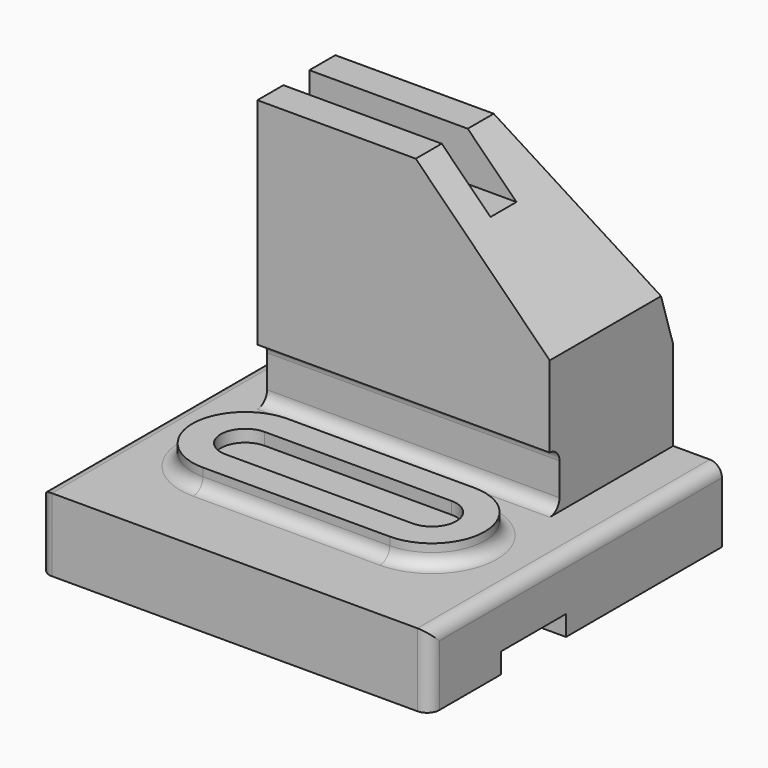
from build123d import *

# Parameters (mm, degrees)
F0_W      = 96
F0_H      = 90
F1_DEPTH  = 18
F2_W      = 72
F2_H      = 38
F4_DEPTH  = 67
F6_DEPTH  = 38
F7_W      = 8
F7_H      = 12
F8_DEPTH  = 51.001
F10_DEPTH = 72.001
F11_W     = 20
F11_H     = 5
F12_DEPTH = 96
F13_W     = 46
F13_H     = 26
F14_DEPTH = 5
F16_DEPTH = 3
F17_W     = 3
F17_H     = 14
F18_DEPTH = 72
F19_R     = 2.99999


# Not quite as in the source:
# - a fillet or chamfer is up to 0.001 mm smaller than in the source, because OpenCascade refuses the exact size


with BuildPart() as f1:
    # F0 (on Top) → F1 (new body)
    with BuildSketch(Plane.XY):
        with Locations((48, 45)):
            Rectangle(F0_W, F0_H)
    extrude(amount=F1_DEPTH)

    # F2 (on face) → F4 (join, through all)
    with BuildSketch(Plane.XY.offset(18)):
        with Locations((48, 71)):
            Rectangle(F2_W, F2_H)
    extrude(amount=F4_DEPTH)

    # F5 (on face) → F6 (cut, through all)
    with BuildSketch(Plane.XZ.offset(-52)):
        Polygon((84, 52), (84, 85), (51, 85), align=None)
    extrude(amount=-F6_DEPTH, mode=Mode.SUBTRACT)

    # F7 (on face) → F8 (cut, through all)
    with BuildSketch(Plane(origin=(12, 0, 0), x_dir=(0, -1, 0), z_dir=(-1, 0, 0))):
        with Locations((-64, 79)):
            Rectangle(F7_W, F7_H)
    extrude(amount=-F8_DEPTH, mode=Mode.SUBTRACT)

    # F9 (on face) → F10 (cut, through all)
    with BuildSketch(Plane(origin=(12, 0, 0), x_dir=(0, -1, 0), z_dir=(-1, 0, 0))):
        Polygon((-90, 40), (-76, 85), (-90, 85), align=None)
    extrude(amount=-F10_DEPTH, mode=Mode.SUBTRACT)

    # F11 (on face) → F12 (cut, through all)
    with BuildSketch(Plane.YZ.offset(96)):
        with Locations((32, 2.5)):
            Rectangle(F11_W, F11_H)
    extrude(amount=-F12_DEPTH, mode=Mode.SUBTRACT)

    # F13 (on face) → F14 (join)
    with BuildSketch(Plane.XY.offset(18)):
        with Locations((48, 31.9999999999)):
            Rectangle(F13_W, F13_H)
        with BuildLine():
            Line((25, 18.9999999999), (25, 44.9999999999))
            ThreePointArc((25, 44.9999999999), (12, 31.9999999999), (25, 18.9999999999))
        make_face()
        with BuildLine():
            ThreePointArc((71, 18.9999999999), (84, 31.9999999999), (71, 44.9999999999))
            Line((71, 44.9999999999), (71, 18.9999999999))
        make_face()
    extrude(amount=F14_DEPTH)

    # F15 (on face) → F16 (cut)
    with BuildSketch(Plane.XY.offset(23)):
        with BuildLine():
            ThreePointArc((71, 25.9999999999), (77, 31.9999999999), (71, 37.9999999999))
            Line((71, 37.9999999999), (71, 25.9999999999))
        make_face()
        Polygon((25, 37.9999999999), (25, 31.9999999999), (25, 25.9999999999), (71, 25.9999999999), (71, 37.9999999999), align=None)
        with BuildLine():
            Line((25, 25.9999999999), (25, 31.9999999999))
            Line((25, 31.9999999999), (25, 37.9999999999))
            ThreePointArc((25, 37.9999999999), (19, 31.9999999999), (25, 25.9999999999))
        make_face()
    extrude(amount=-F16_DEPTH, mode=Mode.SUBTRACT)

    # F17 (on face) → F18 (cut, through all)
    with BuildSketch(Plane.YZ.offset(84)):
        with Locations((53.5, 25)):
            Rectangle(F17_W, F17_H)
    extrude(amount=-F18_DEPTH, mode=Mode.SUBTRACT)

    # F19 (radius 3 in the source; OpenCascade refuses exactly that, so slightly less here)
    f19_edges = [f1.edges().sort_by_distance(p)[0] for p in [
        (48, 55, 18),
        (48, 19, 18),
        (48, 55, 32),
        (96, 45, 18),
        (0, 45, 18),
        (96, 0, 9),
        (0, 0, 9),
    ]]
    fillet(f19_edges, radius=F19_R)


solid = f1.part
